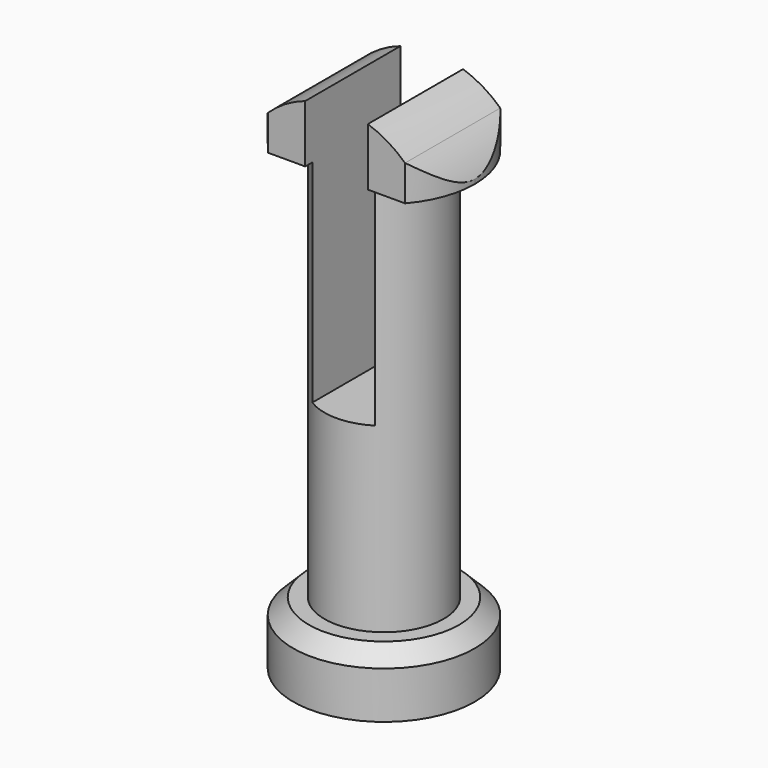
from build123d import *

# Parameters (mm, degrees)
F0_R     = 2.9
F1_DEPTH = 2
F2_R     = 1.9
F3_DEPTH = 12.55
F5_DEPTH = 2
F7_DEPTH = 25
F8_SIZE  = 0.5
F9_DEPTH = 25


# Not quite as in the source:
# - a feature names something its author has since deleted; it is built from what else it names


with BuildPart() as f1:
    # F0 (on Top) → F1 (new body)
    with BuildSketch(Plane.XY):
        with Locations((-52.0645752549, 27.8050955385)):
            Circle(F0_R)
    extrude(amount=F1_DEPTH)

    # F2 (on face) → F3 (join)
    with BuildSketch(Plane.XY.offset(2)):
        with Locations((-52.0645752549, 27.8050955385)):
            Circle(F2_R)
    extrude(amount=F3_DEPTH)

    # F4 (on face) → F5 (join)
    with BuildSketch(Plane.XY.offset(14.55)):
        with BuildLine():
            Line((-52.0645752549, 29.7050955385), (-54.2554654849, 29.7050955385))
            ThreePointArc((-54.2554654849, 29.7050955385), (-54.9645752549, 27.8050955385), (-54.2554654849, 25.9050955385))
            Line((-54.2554654849, 25.9050955385), (-52.0645752549, 25.9050955385))
            ThreePointArc((-52.0645752549, 25.9050955385), (-53.9645752549, 27.8050955385), (-52.0645752549, 29.7050955385))
        make_face()
        with BuildLine():
            ThreePointArc((-50.1645752549, 27.8050955385), (-50.7210723707, 29.1485984228), (-52.0645752549, 29.7050955385))
            ThreePointArc((-52.0645752549, 29.7050955385), (-53.9645752549, 27.8050955385), (-52.0645752549, 25.9050955385))
            ThreePointArc((-52.0645752549, 25.9050955385), (-50.7210723707, 26.4615926542), (-50.1645752549, 27.8050955385))
        make_face()
        with BuildLine():
            ThreePointArc((-49.8736850249, 25.9050955385), (-49.347630126, 26.7910890462), (-49.1645752549, 27.8050955385))
            ThreePointArc((-49.1645752549, 27.8050955385), (-49.347630126, 28.8191020308), (-49.8736850249, 29.7050955385))
            Line((-49.8736850249, 29.7050955385), (-52.0645752549, 29.7050955385))
            ThreePointArc((-52.0645752549, 29.7050955385), (-50.7210723707, 29.1485984228), (-50.1645752549, 27.8050955385))
            ThreePointArc((-50.1645752549, 27.8050955385), (-50.7210723707, 26.4615926542), (-52.0645752549, 25.9050955385))
            Line((-52.0645752549, 25.9050955385), (-49.8736850249, 25.9050955385))
        make_face()
    extrude(amount=F5_DEPTH)

    # F6 (on face) + F5_face1 (on face) → F7 (cut)
    with BuildSketch(Plane.XZ.offset(-25.9050955385)):
        with BuildLine():
            ThreePointArc((-53.0603808121, 16.3889640887), (-52.6208294658, 16.5013745209), (-52.1697451564, 16.55))
            Line((-52.1697451564, 16.55), (-53.0603808121, 16.55))
            Line((-53.0603808121, 16.55), (-53.0603808121, 16.3889640887))
        make_face()
        with BuildLine():
            Line((-51.0603808121, 16.55), (-51.9418670563, 16.55))
            ThreePointArc((-51.9418670563, 16.55), (-51.4955264095, 16.5022285059), (-51.0603808121, 16.3919996636))
            Line((-51.0603808121, 16.3919996636), (-51.0603808121, 16.55))
        make_face()
        with BuildLine():
            Line((-51.0603808121, 16.55), (-51.0603808121, 16.3919996636))
            ThreePointArc((-51.0603808121, 16.3919996636), (-50.428025883, 16.1031256959), (-49.8736850249, 15.6835698131))
            Line((-49.8736850249, 15.6835698131), (-49.8736850249, 16.55))
            Line((-49.8736850249, 16.55), (-51.0603808121, 16.55))
        make_face()
        with BuildLine():
            Line((-49.1058061063, 16.5520446822), (-52.0558061063, 16.5520446822))
            ThreePointArc((-52.0558061063, 16.5520446822), (-51.9988274089, 16.5515334705), (-51.9418670563, 16.55))
            Line((-51.9418670563, 16.55), (-51.0603808121, 16.55))
            Line((-51.0603808121, 16.55), (-49.8736850249, 16.55))
            Line((-49.8736850249, 16.55), (-49.8736850249, 15.6835698131))
            ThreePointArc((-49.8736850249, 15.6835698131), (-49.4281162504, 15.1596303152), (-49.1058061063, 14.5520446822))
            Line((-49.1058061063, 14.5520446822), (-49.1058061063, 16.5520446822))
        make_face()
        with BuildLine():
            Line((-54.2554654849, 16.55), (-54.2554654849, 15.666854741))
            ThreePointArc((-54.2554654849, 15.666854741), (-53.6981031241, 16.0944069239), (-53.0603808121, 16.3889640887))
            Line((-53.0603808121, 16.3889640887), (-53.0603808121, 16.55))
            Line((-53.0603808121, 16.55), (-54.2554654849, 16.55))
        make_face()
        with BuildLine():
            Line((-52.0558061063, 16.5520446822), (-55.0058061063, 16.5520446822))
            Line((-55.0058061063, 16.5520446822), (-55.0058061063, 14.5520446822))
            ThreePointArc((-55.0058061063, 14.5520446822), (-54.6902791648, 15.1495936288), (-54.2554654849, 15.666854741))
            Line((-54.2554654849, 15.666854741), (-54.2554654849, 16.55))
            Line((-54.2554654849, 16.55), (-53.0603808121, 16.55))
            Line((-53.0603808121, 16.55), (-52.1697451564, 16.55))
            ThreePointArc((-52.1697451564, 16.55), (-52.1127848038, 16.5515334705), (-52.0558061063, 16.5520446822))
        make_face()
        Polygon((-52.0645752549, 14.55), (-53.0603808121, 14.55), (-53.0603808121, 7.8), (-51.0603808121, 7.8), (-51.0603808121, 13.8), (-51.0603808121, 14.55), align=None)
    with BuildSketch(Plane(origin=(-52.0645752549, 29.7050955385, 15.55), x_dir=(-1, 0, 0), z_dir=(0, 1, 0))):
        Polygon((-2.19089023, 1), (-2.19089023, -1), (0, -1), (2.19089023, -1), (2.19089023, 1), align=None)
    extrude(amount=-F7_DEPTH, dir=(0, -1, 0), mode=Mode.SUBTRACT)

    # F8
    f8_edges = [f1.edges().sort_by_distance(p)[0] for p in [
        (-54.964575, 27.805096, 2),
    ]]
    chamfer(f8_edges, length=F8_SIZE)

    # F6 (on face) → F9 (cut)
    with BuildSketch(Plane.XZ.offset(-25.9050955385)):
        with BuildLine():
            ThreePointArc((-51.0603808121, 16.3919996636), (-51.4955264095, 16.5022285059), (-51.9418670563, 16.55))
            Line((-51.9418670563, 16.55), (-52.1697451564, 16.55))
            ThreePointArc((-52.1697451564, 16.55), (-52.6208294658, 16.5013745209), (-53.0603808121, 16.3889640887))
            Line((-53.0603808121, 16.3889640887), (-53.0603808121, 14.5520446822))
            Line((-53.0603808121, 14.5520446822), (-53.0603808121, 14.55))
            Line((-53.0603808121, 14.55), (-52.0645752549, 14.55))
            Line((-52.0645752549, 14.55), (-51.0603808121, 14.55))
            Line((-51.0603808121, 14.55), (-51.0603808121, 14.5520446822))
            Line((-51.0603808121, 14.5520446822), (-51.0603808121, 16.3919996636))
        make_face()
        Polygon((-52.0645752549, 14.55), (-53.0603808121, 14.55), (-53.0603808121, 7.8), (-51.0603808121, 7.8), (-51.0603808121, 13.8), (-51.0603808121, 14.55), align=None)
    extrude(amount=-F9_DEPTH, mode=Mode.SUBTRACT)


solid = f1.part
